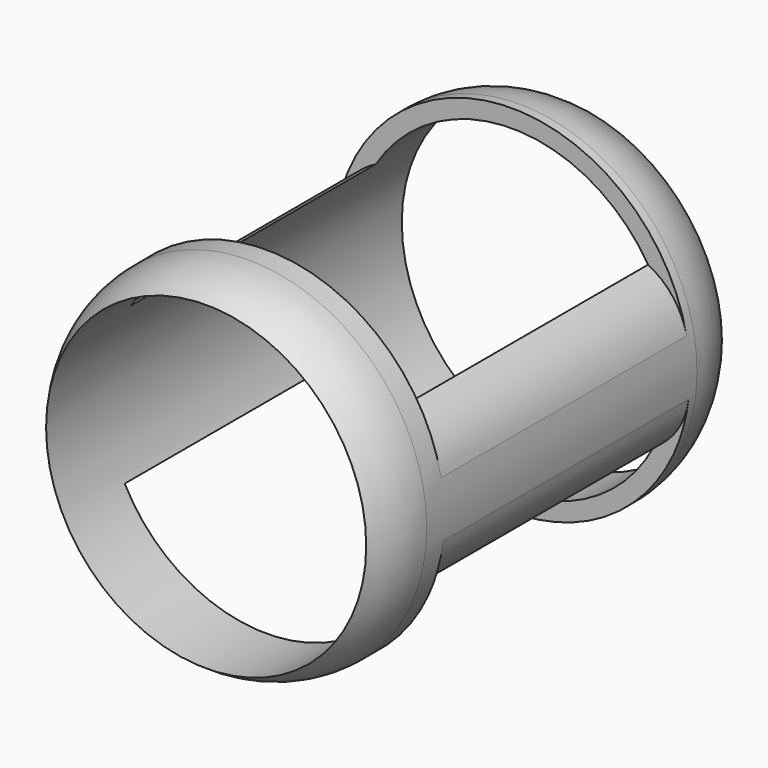
from build123d import *

# Parameters (mm, degrees)
F0_R        = 10
F0_R_2      = 9
F1_DEPTH    = 25
F2_W        = 17.247292446
F2_H        = 6.4440444112
F2_H_2      = 8.7184142321
F3_DEPTH    = 200
F5_T1_DEPTH = 17.247292446


# Not quite as in the source:
# - a fillet or chamfer that OpenCascade refuses, or shapes differently, is made with other operations: its cross-section is extruded or revolved along the edge and cut away or added


with BuildPart() as f1:
    # F0 (on Front) → F1 (new body)
    with BuildSketch(Plane.XZ):
        with Locations((-49.9413348734, 42.8339354694)):
            Circle(F0_R)
        with Locations((-49.9413348734, 42.8339354694)):
            Circle(F0_R_2, mode=Mode.SUBTRACT)
    extrude(amount=F1_DEPTH)

    # F2 (on Right) → F3 (cut)
    with BuildSketch(Plane.YZ):
        with Locations((-12.1299646562, 50.7942251861)):
            Rectangle(F2_W, F2_H)
        with Locations((-12.1299646562, 34.3050556257)):
            Rectangle(F2_W, F2_H_2)
    extrude(amount=-F3_DEPTH, mode=Mode.SUBTRACT)

    # F4: fillet of radius 5 on 2 edges, made by hand

    # F4_s1 → F4_t2 (revolve, cut)
    with BuildSketch(Plane.XY.offset(42.8339354694)):
        with BuildLine():
            ThreePointArc((-39.9413348734, -22), (-40.1979183832, -23.5811388301), (-40.9413348734, -25))
            Line((-40.9413348734, -25), (-39.9413348734, -25))
            Line((-39.9413348734, -25), (-39.9413348734, -22))
        make_face()
    revolve(axis=Axis((-49.9413348734, -25, 42.8339354694), (0, -1, 0)), mode=Mode.SUBTRACT)

    # F4_s3 → F4_t4 (revolve, cut)
    with BuildSketch(Plane.XY.offset(42.8339354694)):
        with BuildLine():
            ThreePointArc((-39.9413348734, -3), (-40.1979183832, -1.4188611699), (-40.9413348734, 0))
            Line((-40.9413348734, 0), (-39.9413348734, 0))
            Line((-39.9413348734, 0), (-39.9413348734, -3))
        make_face()
    revolve(axis=Axis((-49.9413348734, 0, 42.8339354694), (0, -1, 0)), mode=Mode.SUBTRACT)

    # F5: fillet of radius 4 on 4 edges, made by hand

    # F5_s2 → F5_t1 (cut)
    with BuildSketch(Plane.XZ.offset(3.5063184332)):
        with BuildLine():
            ThreePointArc((-59.7567525129, 44.7464146362), (-59.0064973809, 46.4132090316), (-57.5930550064, 47.5722029805))
            Line((-57.5930550064, 47.5722029805), (-58.7475157138, 47.5722029805))
            ThreePointArc((-58.7475157138, 47.5722029805), (-59.3587258299, 46.1973782848), (-59.7567525129, 44.7464146362))
        make_face()
        with BuildLine():
            ThreePointArc((-40.125917234, 44.7464146362), (-40.876172366, 46.4132090316), (-42.2896147405, 47.5722029805))
            Line((-42.2896147405, 47.5722029805), (-41.1351540331, 47.5722029805))
            ThreePointArc((-41.1351540331, 47.5722029805), (-40.5239439169, 46.1973782848), (-40.125917234, 44.7464146362))
        make_face()
        with BuildLine():
            ThreePointArc((-40.0128864724, 41.6398197512), (-40.6400284609, 39.9229099557), (-41.9655070578, 38.6642627418))
            Line((-41.9655070578, 38.6642627418), (-40.8521198719, 38.6642627418))
            ThreePointArc((-40.8521198719, 38.6642627418), (-40.3168159139, 40.1194125284), (-40.0128864724, 41.6398197512))
        make_face()
        with BuildLine():
            ThreePointArc((-59.8697832745, 41.6398197512), (-59.2426412859, 39.9229099557), (-57.9171626891, 38.6642627418))
            Line((-57.9171626891, 38.6642627418), (-59.030549875, 38.6642627418))
            ThreePointArc((-59.030549875, 38.6642627418), (-59.565853833, 40.1194125284), (-59.8697832745, 41.6398197512))
        make_face()
    extrude(amount=F5_T1_DEPTH, mode=Mode.SUBTRACT)


solid = f1.part
